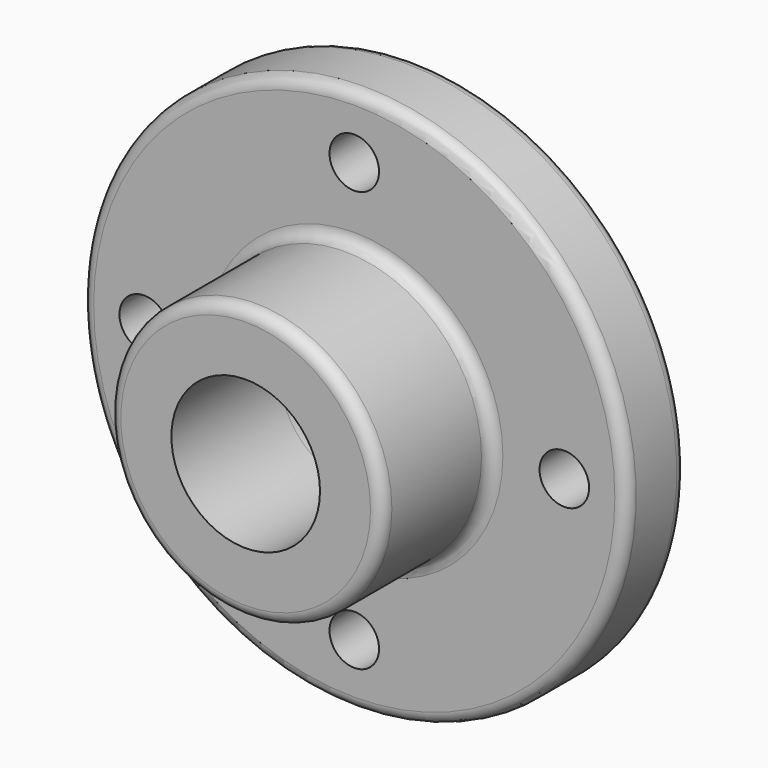
from build123d import *
from build123d import SkipClean  # not in build123d's __all__

# Parameters (mm, degrees)
F0_W            = 19.05
F0_H            = 50.8
F2_R            = 35.052
F2_R_2          = 19.05
F3_DEPTH        = 34.798
F2_R_3          = 6.35
F4_DEPTH        = 19.051
F4_COPIES_COUNT = 4
F5_R            = 3.048
F6_R            = 3.048


# Not quite as in the source:
# - after a boolean that leaves OpenCascade's solid faulty, fix() repairs it
# - a pattern or mirror of a feature is missing from the dataset's text; its kind, count and spacing are read off the source's solid


with BuildPart() as f1:
    # F0 (on Right) → F1 (revolve)
    with BuildSketch(Plane.YZ):
        with Locations((9.525, 44.45)):
            Rectangle(F0_W, F0_H)
    revolve(axis=Axis((0, 24.8311646283, 0), (0, 1, 0)))

    # F2 (on face) → F3 (join)
    with BuildSketch(Plane.XZ):
        Circle(F2_R)
        Circle(F2_R_2, mode=Mode.SUBTRACT)
    with SkipClean():  # cleaning this boolean's faces spoils the solid; the shape is the same uncleaned
        extrude(amount=F3_DEPTH)

    # F2 (on face) → F4 (cut, through all)
    with BuildSketch(Plane.XZ):
        with Locations((0, 53.848)):
            Circle(F2_R_3)
    f4 = extrude(amount=-F4_DEPTH, mode=Mode.SUBTRACT)

    add(f1.part.fix(), mode=Mode.REPLACE)

    # F4_copies: F4 ×4 about axis
    f4_copies_axis = Axis((0, 0, 0), (0, 1, 0))
    for i in range(1, F4_COPIES_COUNT):
        add(f4.rotate(f4_copies_axis, i * 360 / F4_COPIES_COUNT), clean=False, mode=Mode.SUBTRACT)

    # F5
    f5_edges = [f1.edges().sort_by_distance(p)[0] for p in [
        (0, 0, -69.85),
        (0, 19.05, -69.85),
    ]]
    fillet(f5_edges, radius=F5_R)

    # F6
    f6_edges = [f1.edges().sort_by_distance(p)[0] for p in [
        (35.052, -17.399, 0),
        (-35.052, -34.798, 0),
        (-35.052, 0, 0),
    ]]
    fillet(f6_edges, radius=F6_R)


solid = f1.part
